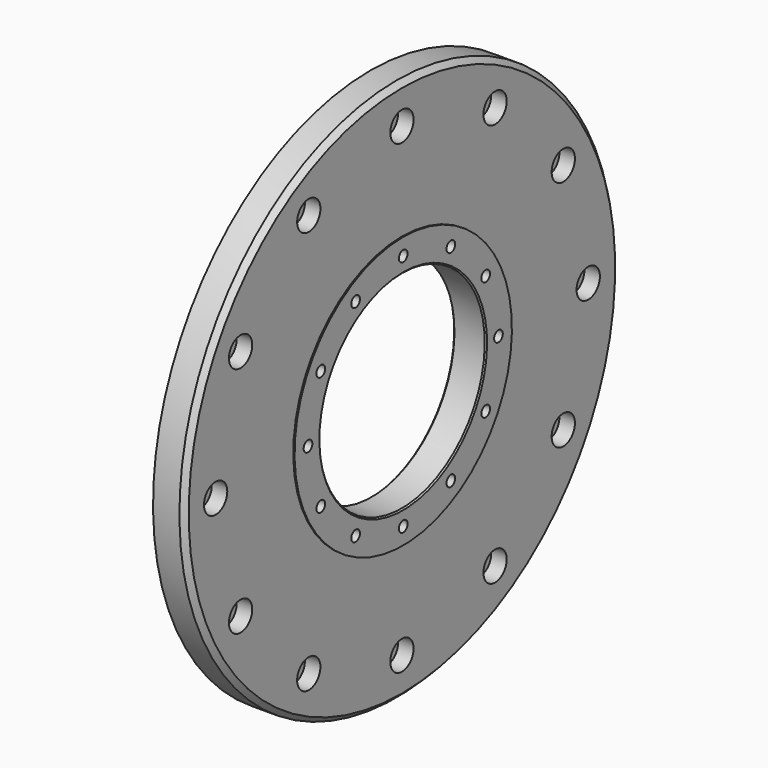
from build123d import *

# Parameters (mm, degrees)
F4_D           = 4.2
F4_CBORE_D     = 8.25
F4_CBORE_DEPTH = 4
F5_D           = 6.3
F5_CBORE_D     = 11.25
F5_CBORE_DEPTH = 6
F6_SIZE        = 2
F7_SIZE        = 0.5


with BuildPart() as f1:
    # F0 (on Front) → F1 (revolve)
    with BuildSketch(Plane.XZ):
        Polygon((-4.6182575495, 105), (-4.6182575495, 80), (-6.6182575495, 80), (-6.6182575495, 74), (-4.6182575495, 74), (-4.6182575495, 40), (8.0817424505, 40), (8.0817424505, 52.5), (7.5817424505, 52.5), (7.5817424505, 105), align=None)
    revolve(axis=Axis((-22.0904547029, 0, 0), (-1, 0, 0)))

    # F4 (through all)
    with Locations(Plane(origin=(-4.6182575495, 0, 0), x_dir=(0, -1, 0), z_dir=(-1, 0, 0))):
        with Locations((0, 46), (23, 39.8371685741), (39.8371685741, 23), (46, 0), (39.8371685741, -23), (23, -39.8371685741), (0, -46), (-23, -39.8371685741), (-46, 0), (-39.8371685741, -23), (-39.8371685741, 23), (-23, 39.8371685741)):
            CounterBoreHole(F4_D / 2, F4_CBORE_D / 2, F4_CBORE_DEPTH)

    # F5 (through all)
    with Locations(Plane.YZ.offset(7.5817424505)):
        with Locations((0, 90), (45, 77.9422863406), (77.9422863406, 45), (90, 0), (77.9422863406, -45), (45, -77.9422863406), (0, -90), (-45, -77.9422863406), (-77.9422863406, -45), (-90, 0), (-77.9422863406, 45), (-45, 77.9422863406)):
            CounterBoreHole(F5_D / 2, F5_CBORE_D / 2, F5_CBORE_DEPTH)

    # F6
    f6_edges = [f1.edges().sort_by_distance(p)[0] for p in [
        (7.581742, 0, -105),
    ]]
    chamfer(f6_edges, length=F6_SIZE)

    # F7
    f7_edges = [f1.edges().sort_by_distance(p)[0] for p in [
        (-6.618258, 0, -80),
        (-6.618258, 0, -74),
        (8.081742, 0, -40),
        (-4.618258, 0, -40),
    ]]
    chamfer(f7_edges, length=F7_SIZE)


solid = f1.part
